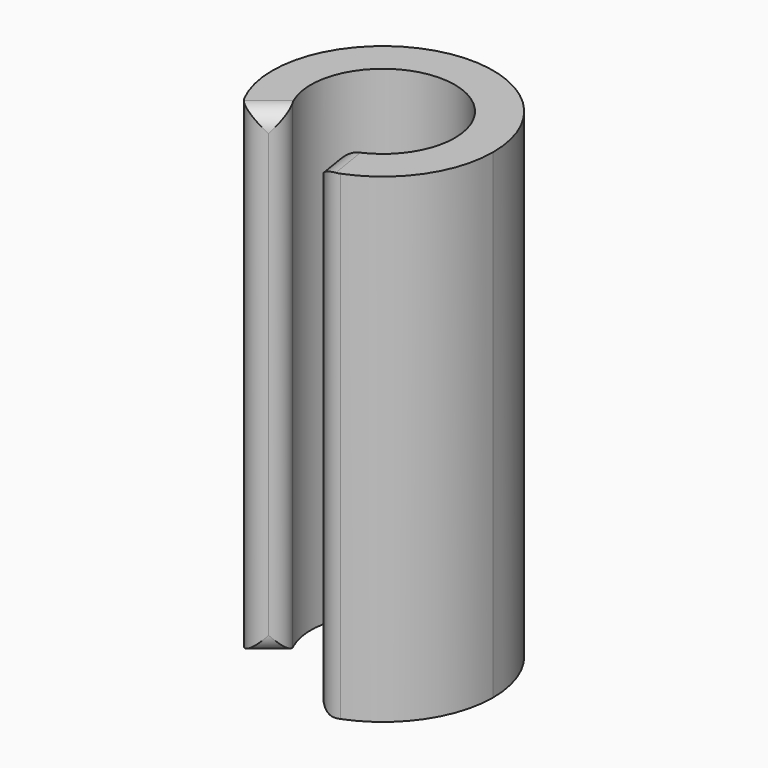
from build123d import *

# Parameters (mm, degrees)
F1_DEPTH = 10
F2_R     = 0.39999


# Not quite as in the source:
# - a fillet or chamfer is up to 0.001 mm smaller than in the source, because OpenCascade refuses the exact size


with BuildPart() as f1:
    # F0 (on Top) → F1 (new body)
    with BuildSketch(Plane.XY):
        with BuildLine():
            ThreePointArc((-1.1635984277, -0.9465932067), (-0.502295908, 1.4133997385), (1.5, 0))
            ThreePointArc((1.5, 0), (1.1417008858, -0.9728921252), (0.2379745502, -1.4810024016))
            Line((0.2379745502, -1.4810024016), (0.3648943103, -2.2708703491))
            ThreePointArc((0.3648943103, -2.2708703491), (1.7506080249, -1.4917679254), (2.3, 0))
            ThreePointArc((2.3, 0), (-0.7701870589, 2.1672129324), (-1.7841842559, -1.4514429169))
            Line((-1.7841842559, -1.4514429169), (-1.1635984277, -0.9465932067))
        make_face()
    extrude(amount=F1_DEPTH)

    # F2 (radius 0.4 in the source; OpenCascade refuses exactly that, so slightly less here)
    f2_edges = [f1.edges().sort_by_distance(p)[0] for p in [
        (-1.784184, -1.451443, 5),
        (-1.163598, -0.946593, 5),
        (-1.473891, -1.199018, 0),
        (-1.473891, -1.199018, 10),
        (0.237975, -1.481002, 5),
        (0.364894, -2.27087, 5),
        (0.301434, -1.875936, 0),
        (0.301434, -1.875936, 10),
    ]]
    fillet(f2_edges, radius=F2_R)


solid = f1.part
